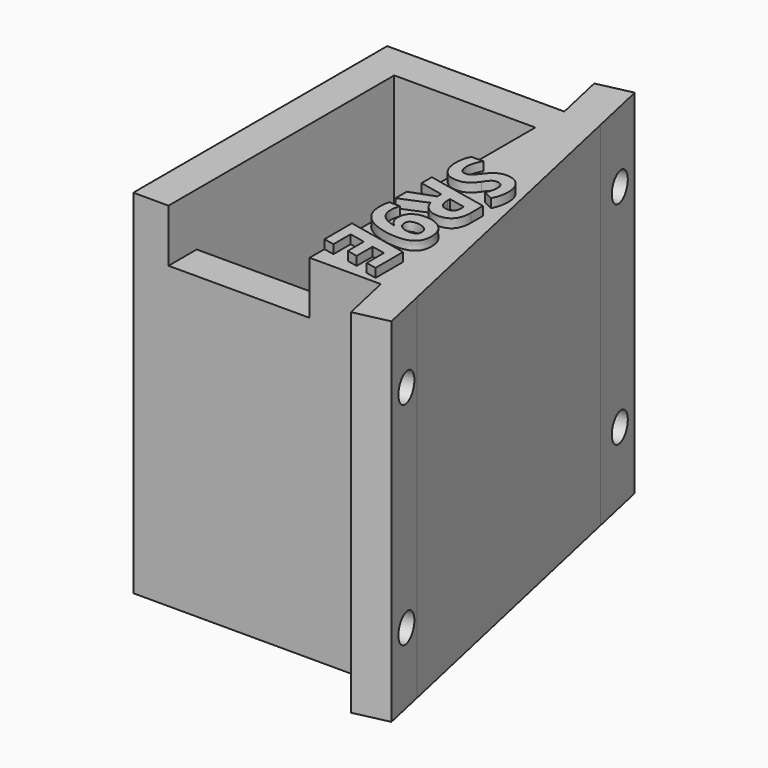
from build123d import *

# Parameters (mm, degrees)
F0_W         = 25.4
F0_H         = 44.45
F1_DEPTH     = 63.5
F2_W         = 25.4
F2_H         = 6.35
F3_DEPTH     = 9.525
F4_TEXT_SIZE = 15.5076341031
F5_DEPTH     = 1.5875
F6_R         = 2.55
F7_DEPTH     = 25.4
F8_R         = 2.55
F9_DEPTH     = 25.4


# Not quite as in the source:
# - a length typed as a fraction of an inch, garbled in the dataset ("3 / 203.2 mm" for 3/8 in), is restored
# - Text() gives the source's letters only with a copy of the font that has no kerning and outlines rounded to 1/6400 em; it was checked with that copy


with BuildPart() as f1:
    # F0 (on Top) → F1 (new body)
    with BuildSketch(Plane.XY):
        Polygon((-6.35, 50.8), (-6.35, -6.35), (31.75, -6.35), (38.2204219002, -6.35), (40.282009223, -15.6492194678), (46.4814888682, -14.2748279193), (44.7245968161, -6.35), (32.0547468461, 50.8), (29.6884642526, 61.4736110163), (23.4889846074, 60.0992194678), (25.5505719302, 50.8), align=None)
        with Locations((12.7, 22.225)):
            Rectangle(F0_W, F0_H, mode=Mode.SUBTRACT)
    extrude(amount=F1_DEPTH)

    # F2 (on face) → F3 (cut)
    with BuildSketch(Plane.XY.offset(63.5)):
        with Locations((12.7, -3.175)):
            Rectangle(F2_W, F2_H)
    extrude(amount=-F3_DEPTH, mode=Mode.SUBTRACT)

    # F4 (on face) → F5 (join)
    with BuildSketch(Plane.XY.offset(63.5)):
        with Locations(Location((25.4, 29.7924797316), (0, 0, -90))):
            Text('SR9E', F4_TEXT_SIZE, font='Open Sans', font_style=FontStyle.BOLDITALIC, text_align=(TextAlign.LEFT, TextAlign.BOTTOM))
    extrude(amount=F5_DEPTH)

    # F6 (on face) → F7 (cut)
    with BuildSketch(Plane(origin=(35.0881309651, 7.7788513571, 0), x_dir=(0.2164396139, -0.9762960071, 0), z_dir=(-0.9762960071, -0.2164396139, 0))):
        with Locations((19.2343930058, 50.8)):
            Circle(F6_R)
        with Locations((19.2343930058, 12.7)):
            Circle(F6_R)
    extrude(amount=-F7_DEPTH, mode=Mode.SUBTRACT)

    # F8 (on face) → F9 (cut)
    with BuildSketch(Plane(origin=(35.0881309651, 7.7788513571, 0), x_dir=(0.2164396139, -0.9762960071, 0), z_dir=(-0.9762960071, -0.2164396139, 0))):
        with Locations((-48.8281812372, 50.8)):
            Circle(F8_R)
        with Locations((-48.8281812372, 12.7)):
            Circle(F8_R)
    extrude(amount=-F9_DEPTH, mode=Mode.SUBTRACT)


solid = f1.part
